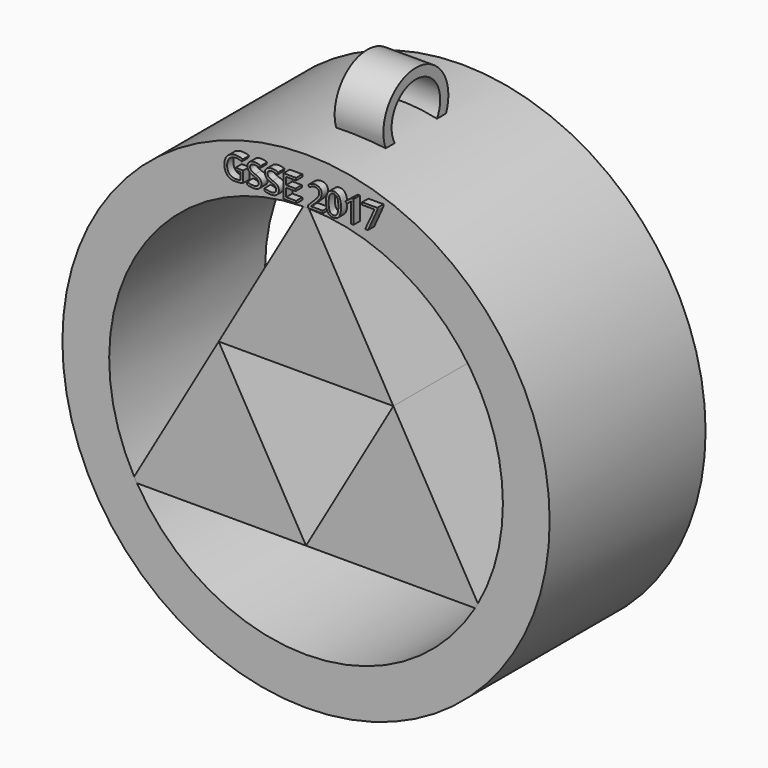
from build123d import *

# Parameters (mm, degrees)
F0_R         = 31.75
F1_DEPTH     = 25.4
F2_DEPTH     = 25.4
F3_R         = 5.2911855335
F3_R_2       = 3.9599835796
F4_DEPTH     = 6.35
F5_TEXT_SIZE = 4.1368915441
F6_DEPTH     = 26.416


# Not quite as in the source:
# - Text() gives the source's letters only with a copy of the font that has no kerning and outlines rounded to 1/6400 em; it was checked with that copy


with BuildPart() as f1:
    # F0 (on Front) → F1 (new body)
    with BuildSketch(Plane.XZ):
        with Locations((-5.0221197307, -1.6293748049)):
            Circle(F0_R)
        with BuildLine():
            ThreePointArc((-4.6559703131, 24.0231625016), (13.247805748, 16.381637345), (20.6330305448, -1.6293748049))
            ThreePointArc((20.6330305448, -1.6293748049), (19.805605934, -8.0924061352), (17.3767039571, -14.1385487609))
            ThreePointArc((17.3767039571, -14.1385487609), (17.1958921458, -14.4569499427), (17.0105545394, -14.7727381554))
            ThreePointArc((17.0105545394, -14.7727381554), (-5.0221197307, -27.2845250804), (-27.0547940009, -14.7727381554))
            ThreePointArc((-27.0547940009, -14.7727381554), (-27.2401316072, -14.4569499427), (-27.4209434185, -14.1385487609))
            ThreePointArc((-27.4209434185, -14.1385487609), (-27.2401316072, 11.1982003328), (-5.3882691484, 24.0231625016))
            ThreePointArc((-5.3882691484, 24.0231625016), (-5.0221197307, 24.0257754706), (-4.6559703131, 24.0231625016))
        make_face(mode=Mode.SUBTRACT)
    extrude(amount=F1_DEPTH)

    # F3 (on Right) → F4 (join)
    with BuildSketch(Plane.YZ):
        with Locations((-13.7844085693, 31.6802300513)):
            Circle(F3_R)
        with Locations((-13.7844085693, 31.6802300513)):
            Circle(F3_R_2, mode=Mode.SUBTRACT)
    extrude(amount=-F4_DEPTH)

    # F5 (on Front) → F6 (join)
    with BuildSketch(Plane.XZ):
        with Locations((-15.1066724211, 24.7309445404)):
            Text('GSSE 2017', F5_TEXT_SIZE, font='Open Sans', text_align=(TextAlign.LEFT, TextAlign.BOTTOM))
    extrude(amount=F6_DEPTH)


with BuildPart() as f2:
    # F0 (on Front) → F2 (new body)
    with BuildSketch(Plane.XZ):
        with BuildLine():
            Line((6.360366822, 4.9423068704), (-4.6559703131, 24.0231625016))
            ThreePointArc((-4.6559703131, 24.0231625016), (-5.0221197307, 24.0257754706), (-5.3882691484, 24.0231625016))
            Line((-5.3882691484, 24.0231625016), (-16.4046062834, 4.9423068704))
            Line((-16.4046062834, 4.9423068704), (6.360366822, 4.9423068704))
        make_face()
    extrude(amount=F2_DEPTH)


with BuildPart() as f2b:
    # F0 (on Front) → F2, piece 2 (new body)
    with BuildSketch(Plane.XZ):
        with BuildLine():
            ThreePointArc((17.0105545394, -14.7727381554), (17.1958921458, -14.4569499427), (17.3767039571, -14.1385487609))
            Line((17.3767039571, -14.1385487609), (6.360366822, 4.9423068704))
            Line((6.360366822, 4.9423068704), (-5.0221197307, -14.7727381554))
            Line((-5.0221197307, -14.7727381554), (17.0105545394, -14.7727381554))
        make_face()
    extrude(amount=F2_DEPTH)


with BuildPart() as f2c:
    # F0 (on Front) → F2, piece 3 (new body)
    with BuildSketch(Plane.XZ):
        with BuildLine():
            Line((-16.4046062834, 4.9423068704), (-27.4209434185, -14.1385487609))
            ThreePointArc((-27.4209434185, -14.1385487609), (-27.2401316072, -14.4569499427), (-27.0547940009, -14.7727381554))
            Line((-27.0547940009, -14.7727381554), (-5.0221197307, -14.7727381554))
            Line((-5.0221197307, -14.7727381554), (-16.4046062834, 4.9423068704))
        make_face()
    extrude(amount=F2_DEPTH)


solid = Compound([f1.part, f2.part, f2b.part, f2c.part])
